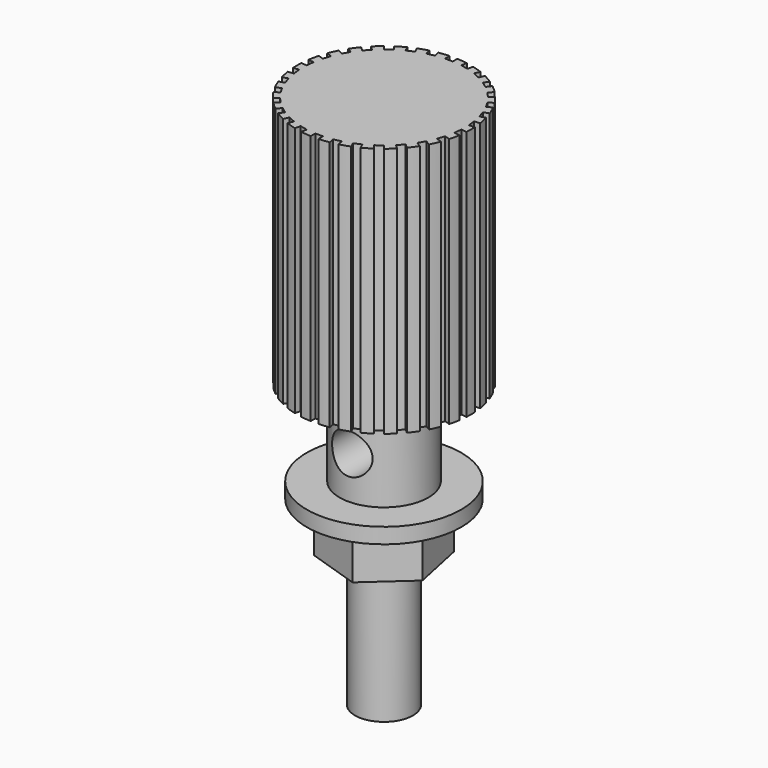
from build123d import *

# Parameters (mm, degrees)
F0_R      = 4
F1_DEPTH  = 0.8
F2_R      = 2.3
F3_DEPTH  = 4.5
F4_R      = 4.5
F5_DEPTH  = 13
F6_R      = 1.5
F7_DEPTH  = 9.4
F8_R      = 1.05
F9_DEPTH  = 12.5
F10_W     = 0.4
F10_H     = 0.6
F11_DEPTH = 25
F12_COUNT = 30
F15_DEPTH = 2.5


with BuildPart() as f1:
    # F0 (on Top) → F1 (new body)
    with BuildSketch(Plane.XY):
        Circle(F0_R)
    extrude(amount=F1_DEPTH)

    # F2 (on face) → F3 (join)
    with BuildSketch(Plane.XY.offset(0.8)):
        Circle(F2_R)
    extrude(amount=F3_DEPTH)

    # F4 (on face) → F5 (join)
    with BuildSketch(Plane.XY.offset(5.3)):
        Circle(F4_R)
    extrude(amount=F5_DEPTH)

    # F6 (on face) → F7 (join)
    with BuildSketch(Plane(origin=(0, 0, 0), x_dir=(1, 0, 0), z_dir=(0, 0, -1))):
        Circle(F6_R)
    extrude(amount=F7_DEPTH)

    # F8 (on Front) → F9 (cut, symmetric)
    with BuildSketch(Plane.XZ):
        with Locations((0, 3)):
            Circle(F8_R)
    extrude(amount=F9_DEPTH, both=True, mode=Mode.SUBTRACT)


with BuildPart() as f11:
    # F10 (on face) → F11 (new body)
    with BuildSketch(Plane.XY.offset(18.3)):
        with Locations((0, 4.5)):
            Rectangle(F10_W, F10_H)
    extrude(amount=-F11_DEPTH)


with BuildPart() as f12_1:
    # F12: instance of F11
    add(f11.part.rotate(Axis((0, 0, 18.3), (0, 0, 1)), 1 * 360 / F12_COUNT))


with BuildPart() as f12_2:
    # F12: instance of F11
    add(f11.part.rotate(Axis((0, 0, 18.3), (0, 0, 1)), 2 * 360 / F12_COUNT))


with BuildPart() as f12_3:
    # F12: instance of F11
    add(f11.part.rotate(Axis((0, 0, 18.3), (0, 0, 1)), 3 * 360 / F12_COUNT))


with BuildPart() as f12_4:
    # F12: instance of F11
    add(f11.part.rotate(Axis((0, 0, 18.3), (0, 0, 1)), 4 * 360 / F12_COUNT))


with BuildPart() as f12_5:
    # F12: instance of F11
    add(f11.part.rotate(Axis((0, 0, 18.3), (0, 0, 1)), 5 * 360 / F12_COUNT))


with BuildPart() as f12_6:
    # F12: instance of F11
    add(f11.part.rotate(Axis((0, 0, 18.3), (0, 0, 1)), 6 * 360 / F12_COUNT))


with BuildPart() as f12_7:
    # F12: instance of F11
    add(f11.part.rotate(Axis((0, 0, 18.3), (0, 0, 1)), 7 * 360 / F12_COUNT))


with BuildPart() as f12_8:
    # F12: instance of F11
    add(f11.part.rotate(Axis((0, 0, 18.3), (0, 0, 1)), 8 * 360 / F12_COUNT))


with BuildPart() as f12_9:
    # F12: instance of F11
    add(f11.part.rotate(Axis((0, 0, 18.3), (0, 0, 1)), 9 * 360 / F12_COUNT))


with BuildPart() as f12_10:
    # F12: instance of F11
    add(f11.part.rotate(Axis((0, 0, 18.3), (0, 0, 1)), 10 * 360 / F12_COUNT))


with BuildPart() as f12_11:
    # F12: instance of F11
    add(f11.part.rotate(Axis((0, 0, 18.3), (0, 0, 1)), 11 * 360 / F12_COUNT))


with BuildPart() as f12_12:
    # F12: instance of F11
    add(f11.part.rotate(Axis((0, 0, 18.3), (0, 0, 1)), 12 * 360 / F12_COUNT))


with BuildPart() as f12_13:
    # F12: instance of F11
    add(f11.part.rotate(Axis((0, 0, 18.3), (0, 0, 1)), 13 * 360 / F12_COUNT))


with BuildPart() as f12_14:
    # F12: instance of F11
    add(f11.part.rotate(Axis((0, 0, 18.3), (0, 0, 1)), 14 * 360 / F12_COUNT))


with BuildPart() as f12_15:
    # F12: instance of F11
    add(f11.part.rotate(Axis((0, 0, 18.3), (0, 0, 1)), 15 * 360 / F12_COUNT))


with BuildPart() as f12_16:
    # F12: instance of F11
    add(f11.part.rotate(Axis((0, 0, 18.3), (0, 0, 1)), 16 * 360 / F12_COUNT))


with BuildPart() as f12_17:
    # F12: instance of F11
    add(f11.part.rotate(Axis((0, 0, 18.3), (0, 0, 1)), 17 * 360 / F12_COUNT))


with BuildPart() as f12_18:
    # F12: instance of F11
    add(f11.part.rotate(Axis((0, 0, 18.3), (0, 0, 1)), 18 * 360 / F12_COUNT))


with BuildPart() as f12_19:
    # F12: instance of F11
    add(f11.part.rotate(Axis((0, 0, 18.3), (0, 0, 1)), 19 * 360 / F12_COUNT))


with BuildPart() as f12_20:
    # F12: instance of F11
    add(f11.part.rotate(Axis((0, 0, 18.3), (0, 0, 1)), 20 * 360 / F12_COUNT))


with BuildPart() as f12_21:
    # F12: instance of F11
    add(f11.part.rotate(Axis((0, 0, 18.3), (0, 0, 1)), 21 * 360 / F12_COUNT))


with BuildPart() as f12_22:
    # F12: instance of F11
    add(f11.part.rotate(Axis((0, 0, 18.3), (0, 0, 1)), 22 * 360 / F12_COUNT))


with BuildPart() as f12_23:
    # F12: instance of F11
    add(f11.part.rotate(Axis((0, 0, 18.3), (0, 0, 1)), 23 * 360 / F12_COUNT))


with BuildPart() as f12_24:
    # F12: instance of F11
    add(f11.part.rotate(Axis((0, 0, 18.3), (0, 0, 1)), 24 * 360 / F12_COUNT))


with BuildPart() as f12_25:
    # F12: instance of F11
    add(f11.part.rotate(Axis((0, 0, 18.3), (0, 0, 1)), 25 * 360 / F12_COUNT))


with BuildPart() as f12_26:
    # F12: instance of F11
    add(f11.part.rotate(Axis((0, 0, 18.3), (0, 0, 1)), 26 * 360 / F12_COUNT))


with BuildPart() as f12_27:
    # F12: instance of F11
    add(f11.part.rotate(Axis((0, 0, 18.3), (0, 0, 1)), 27 * 360 / F12_COUNT))


with BuildPart() as f12_28:
    # F12: instance of F11
    add(f11.part.rotate(Axis((0, 0, 18.3), (0, 0, 1)), 28 * 360 / F12_COUNT))


with BuildPart() as f12_29:
    # F12: instance of F11
    add(f11.part.rotate(Axis((0, 0, 18.3), (0, 0, 1)), 29 * 360 / F12_COUNT))


with BuildPart() as f1_1:
    add(f1.part)

    # F13: cut F12_1, F12_2, F12_3, F12_4, F12_5, F12_6, F12_7, F12_8, F12_9, F12_10, F12_11, F12_12, F12_13, F12_14, F12_15, F12_16, F12_17, F12_18, F12_19, F12_20, F12_21, F12_22, F12_23, F12_24, F12_25, F12_26, F12_27, F12_28, F12_29, F11
    add(f12_1.part, mode=Mode.SUBTRACT)
    add(f12_2.part, mode=Mode.SUBTRACT)
    add(f12_3.part, mode=Mode.SUBTRACT)
    add(f12_4.part, mode=Mode.SUBTRACT)
    add(f12_5.part, mode=Mode.SUBTRACT)
    add(f12_6.part, mode=Mode.SUBTRACT)
    add(f12_7.part, mode=Mode.SUBTRACT)
    add(f12_8.part, mode=Mode.SUBTRACT)
    add(f12_9.part, mode=Mode.SUBTRACT)
    add(f12_10.part, mode=Mode.SUBTRACT)
    add(f12_11.part, mode=Mode.SUBTRACT)
    add(f12_12.part, mode=Mode.SUBTRACT)
    add(f12_13.part, mode=Mode.SUBTRACT)
    add(f12_14.part, mode=Mode.SUBTRACT)
    add(f12_15.part, mode=Mode.SUBTRACT)
    add(f12_16.part, mode=Mode.SUBTRACT)
    add(f12_17.part, mode=Mode.SUBTRACT)
    add(f12_18.part, mode=Mode.SUBTRACT)
    add(f12_19.part, mode=Mode.SUBTRACT)
    add(f12_20.part, mode=Mode.SUBTRACT)
    add(f12_21.part, mode=Mode.SUBTRACT)
    add(f12_22.part, mode=Mode.SUBTRACT)
    add(f12_23.part, mode=Mode.SUBTRACT)
    add(f12_24.part, mode=Mode.SUBTRACT)
    add(f12_25.part, mode=Mode.SUBTRACT)
    add(f12_26.part, mode=Mode.SUBTRACT)
    add(f12_27.part, mode=Mode.SUBTRACT)
    add(f12_28.part, mode=Mode.SUBTRACT)
    add(f12_29.part, mode=Mode.SUBTRACT)
    add(f11.part, mode=Mode.SUBTRACT)

    # F14 (on face) → F15 (join)
    with BuildSketch(Plane(origin=(0, 0, 0), x_dir=(1, 0, 0), z_dir=(0, 0, -1))):
        Polygon((-2.6927305179, -0.8780481684), (-0.5859532394, -2.7709971182), (2.1067772785, -1.8929489498), (2.6927305179, 0.8780481684), (0.5859532394, 2.7709971182), (-2.1067772785, 1.8929489498), align=None)
    extrude(amount=F15_DEPTH)


solid = f1_1.part
